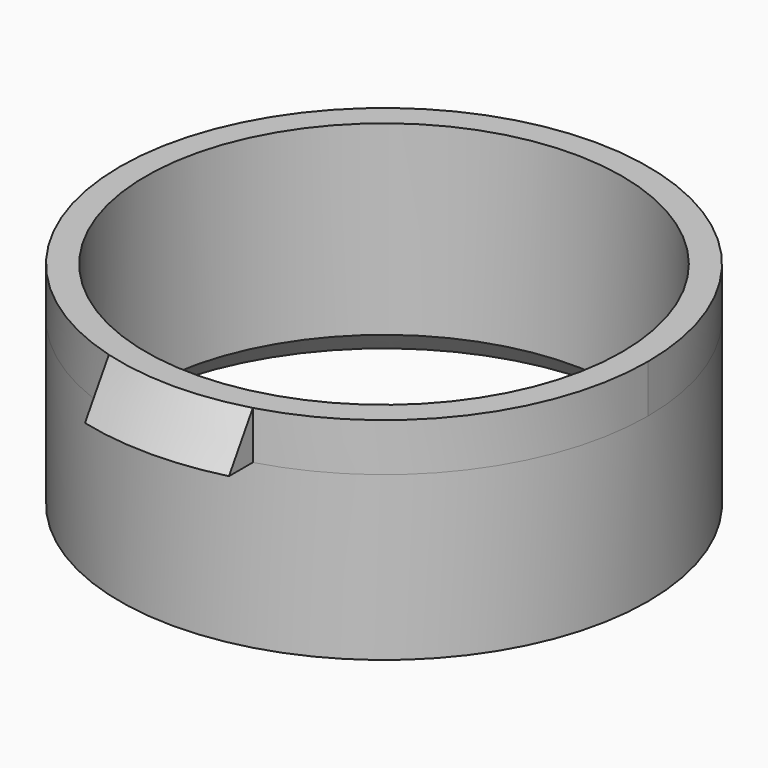
from build123d import *
from build123d import SkipClean  # not in build123d's __all__

# Parameters (mm, degrees)
F0_R     = 27.5
F0_R_2   = 24.8
F1_DEPTH = 22
F4_W     = 80.197357
F4_H     = 91.318484
F5_DEPTH = 42.3
F6_SIZE  = 2.6


with BuildPart() as f1:
    # F0 (on Top) → F1 (new body)
    with BuildSketch(Plane.XY):
        Circle(F0_R)
        Circle(F0_R_2, mode=Mode.SUBTRACT)
    extrude(amount=F1_DEPTH)

    # F2 (on Right) → F3 (revolve)
    with BuildSketch(Plane.YZ):
        Polygon((-30.5, 17), (-27.5, 17), (-27.5, 22), align=None)
    revolve(axis=Axis((0, 0, 0), (0, 0, -1)))

    # F4 (on Top) → F5 (cut)
    with BuildSketch(Plane.XY):
        with Locations((-0.965879, 0.658857)):
            Rectangle(F4_W, F4_H)
        with BuildLine():
            Line((-7.5, 26.457513), (-7.5, 35.975846))
            Line((-7.5, 35.975846), (7.5, 35.975846))
            Line((7.5, 35.975846), (7.5, 26.457513))
            ThreePointArc((7.5, 26.457513), (21.937411, 16.583124), (27.5, 0))
            ThreePointArc((27.5, 0), (21.937411, -16.583124), (7.5, -26.457513))
            Line((7.5, -26.457513), (7.5, -34.024154))
            Line((7.5, -34.024154), (-7.5, -34.024154))
            Line((-7.5, -34.024154), (-7.5, -26.457513))
            ThreePointArc((-7.5, -26.457513), (-27.5, 0), (-7.5, 26.457513))
        make_face(mode=Mode.SUBTRACT)
    with SkipClean():  # cleaning this boolean's faces spoils the solid; the shape is the same uncleaned
        extrude(amount=F5_DEPTH, mode=Mode.SUBTRACT)

    # F6
    f6_edges = [f1.edges().sort_by_distance(p)[0] for p in [
        (-24.8, 0, 0),
    ]]
    chamfer(f6_edges, length=F6_SIZE)


solid = f1.part
